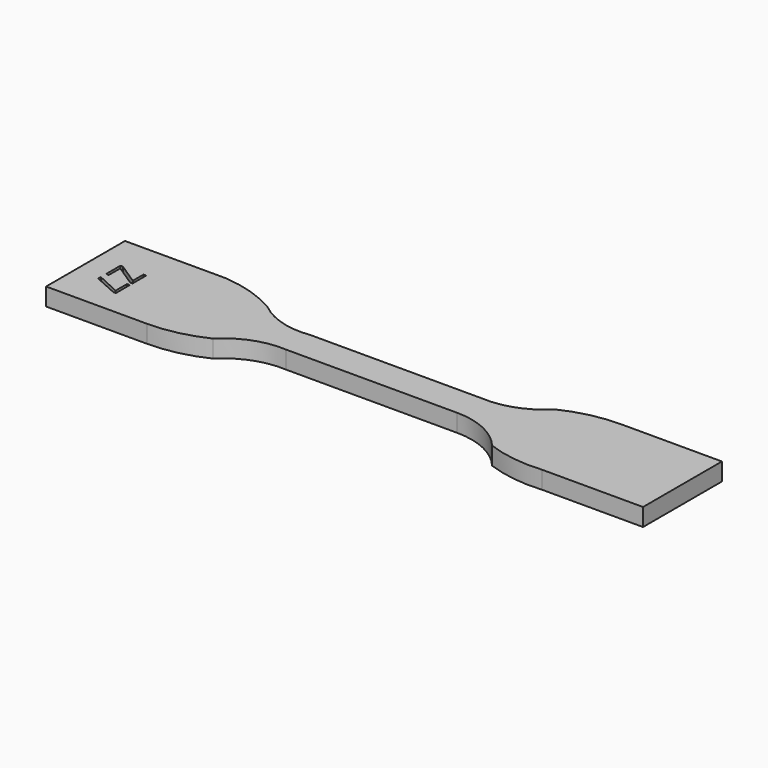
from build123d import *

# Parameters (mm, degrees)
F1_DEPTH     = 3.4
F2_TEXT_SIZE = 7.0564552314
F3_DEPTH     = 1


# Not quite as in the source:
# - Text() gives the source's letters only with a copy of the font that has no kerning and outlines rounded to 1/6400 em; it was checked with that copy


with BuildPart() as f1:
    # F0 (on Top) → F1 (new body)
    with BuildSketch(Plane.XY):
        with BuildLine():
            Line((-14.4320548165, 19.7811394548), (-33.8720548165, 19.7811394548))
            Line((-33.8720548165, 19.7811394548), (-33.8720548165, 0.7811394548))
            Line((-33.8720548165, 0.7811394548), (-14.4320548165, 0.7811394548))
            ThreePointArc((-14.4320548165, 0.7811394548), (-8.9053122052, 1.3996892086), (-3.6520548165, 3.2247301661))
            ThreePointArc((-3.6520548165, 3.2247301661), (1.3014698263, 6.4128780055), (7.1279451835, 7.2811394548))
            Line((7.1279451835, 7.2811394548), (40.1279451835, 7.2811394548))
            ThreePointArc((40.1279451835, 7.2811394548), (46.0837574042, 5.9511158081), (50.9079451835, 2.2137538538))
            ThreePointArc((50.9079451835, 2.2137538538), (56.2191047011, 0.9041953221), (61.6879451835, 0.7811394548))
            Line((61.6879451835, 0.7811394548), (81.1279451835, 0.7811394548))
            Line((81.1279451835, 0.7811394548), (81.1279451835, 19.7811394548))
            Line((81.1279451835, 19.7811394548), (61.6879451835, 19.7811394548))
            ThreePointArc((61.6879451835, 19.7811394548), (56.1612025723, 19.162589701), (50.9079451835, 17.3375487435))
            ThreePointArc((50.9079451835, 17.3375487435), (45.9544205407, 14.1494009041), (40.1279451835, 13.2811394548))
            Line((40.1279451835, 13.2811394548), (7.1279451835, 13.2811394548))
            ThreePointArc((7.1279451835, 13.2811394548), (1.4167452884, 13.6925537245), (-3.6520548165, 16.3560723447))
            ThreePointArc((-3.6520548165, 16.3560723447), (-8.8458057958, 18.686276846), (-14.4320548165, 19.7811394548))
        make_face()
    extrude(amount=F1_DEPTH)

    # F2 (on face) → F3 (cut)
    with BuildSketch(Plane.XY.offset(3.4)):
        with Locations(Location((-29.3720550835, 13.353464842), (0, 0, -90))):
            Text('Z7', F2_TEXT_SIZE, font='Open Sans', text_align=(TextAlign.LEFT, TextAlign.BOTTOM))
    extrude(amount=-F3_DEPTH, mode=Mode.SUBTRACT)


solid = f1.part
